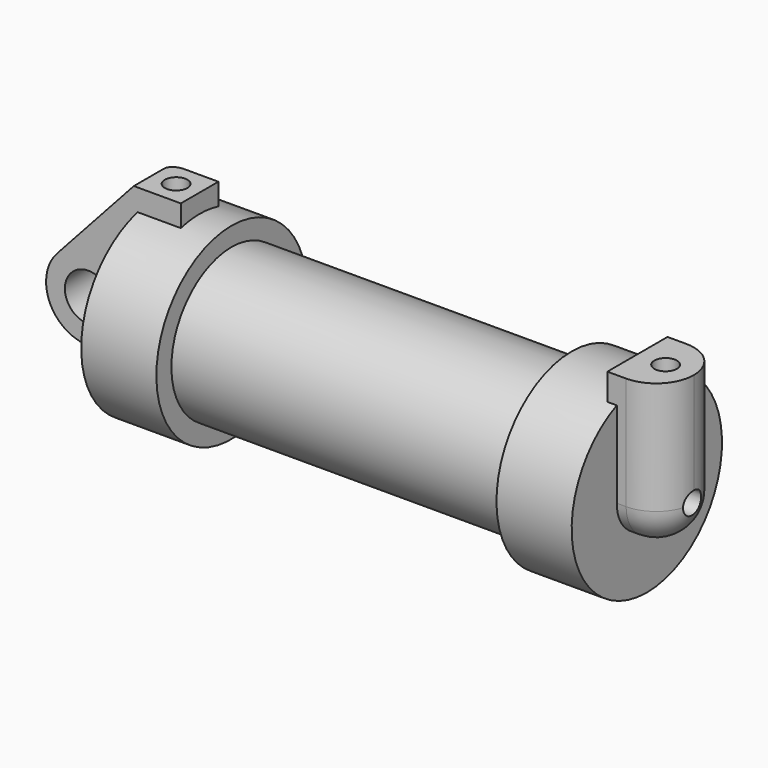
from build123d import *

# Parameters (mm, degrees)
F0_W          = 5.842
F0_H          = 12.7
F0_R          = 3.175
F2_DEPTH      = 3.175
F3_R          = 1.524
F4_DEPTH      = 6.35
F4_DEPTH_BACK = 1.27
F5_R          = 1.524
F6_DEPTH      = 10.414
F7_R          = 1.524
F8_DEPTH      = 17.78
F9_DEPTH      = 56.134
F10_R         = 1.27
F11_T1_DEPTH  = 27.94
F11_T4_ANGLE  = 180


# Not quite as in the source:
# - a fillet or chamfer that OpenCascade refuses, or shapes differently, is made with other operations: its cross-section is extruded or revolved along the edge and cut away or added


with BuildPart() as f1:
    # F0 (on Front) → F1 (revolve)
    with BuildSketch(Plane.XZ):
        Polygon((5.842, 12.7), (5.842, 0), (66.294, 0), (66.294, 12.7), (56.134, 12.7), (56.134, 10.16), (10.16, 10.16), (10.16, 12.7), align=None)
        with Locations((2.921, 6.35)):
            Rectangle(F0_W, F0_H)
    revolve(axis=Axis((33.147, 0, 0), (-1, 0, 0)))

    # F0 (on Front) → F2 (join, symmetric)
    with BuildSketch(Plane.XZ):
        with BuildLine():
            Line((-0.9398, 0), (0, 0))
            Line((0, 0), (0, 12.7))
            Line((0, 12.7), (5.842, 12.7))
            Line((5.842, 12.7), (5.842, 15.24))
            Line((5.842, 15.24), (-0.508, 15.24))
            Line((-0.508, 15.24), (-10.8806298187, 3.8475430269))
            ThreePointArc((-10.8806298187, 3.8475430269), (-4.5919612295, 5.3297205562), (-0.9398, 0))
        make_face()
        with Locations((2.921, 6.35)):
            Rectangle(F0_W, F0_H)
        with BuildLine():
            Line((5.842, 0), (0, 0))
            Line((0, 0), (-0.9398, 0))
            ThreePointArc((-0.9398, 0), (-3.1957909266, -4.5493385486), (-8.1826630726, -5.5069827884))
            Line((-8.1826630726, -5.5069827884), (5.842, -9.398))
            Line((5.842, -9.398), (5.842, 0))
        make_face()
        with BuildLine():
            ThreePointArc((-8.1826630726, -5.5069827884), (-3.1957909266, -4.5493385486), (-0.9398, 0))
            ThreePointArc((-0.9398, 0), (-4.5919612295, 5.3297205562), (-10.8806298187, 3.8475430269))
            ThreePointArc((-10.8806298187, 3.8475430269), (-12.1459778134, -1.5837270034), (-8.1826630726, -5.5069827884))
        make_face()
        with Locations((-6.6548, 0)):
            Circle(F0_R, mode=Mode.SUBTRACT)
    extrude(amount=F2_DEPTH, both=True)

    # F3 (on face) → F4 (join, two sides)
    with BuildSketch(Plane.YZ.offset(66.294)) as f4_sk:
        with BuildLine():
            ThreePointArc((-5.08, 0), (0, -5.08), (5.08, 0))
            ThreePointArc((5.08, 0), (0, 5.08), (-5.08, 0))
        make_face()
        Circle(F3_R, mode=Mode.SUBTRACT)
        with BuildLine():
            ThreePointArc((-5.08, 0), (0, 5.08), (5.08, 0))
            Line((5.08, 0), (5.08, 15.24))
            Line((5.08, 15.24), (-5.08, 15.24))
            Line((-5.08, 15.24), (-5.08, 0))
        make_face()
    extrude(amount=F4_DEPTH)
    extrude(f4_sk.sketch, amount=-F4_DEPTH_BACK)

    # F5 (on face) → F6 (cut)
    with BuildSketch(Plane.XY.offset(15.24)):
        with Locations((68.834, 0)):
            Circle(F5_R)
    extrude(amount=-F6_DEPTH, mode=Mode.SUBTRACT)

    # F7 (on face) → F8 (cut)
    with BuildSketch(Plane.XY.offset(15.24)):
        with Locations((2.667, 0)):
            Circle(F7_R)
    extrude(amount=-F8_DEPTH, mode=Mode.SUBTRACT)

    # F9 (cut, through all): a face of the model
    f9_faces = [f1.faces().sort_by_distance(p)[0] for p in [
        (66.294, 0, 0),
    ]]
    extrude(f9_faces, amount=-F9_DEPTH, mode=Mode.SUBTRACT)

    # F10
    f10_edges = [f1.edges().sort_by_distance(p)[0] for p in [
        (-12.145978, 3.175, -1.583727),
        (-5.694315, 3.175, 9.543772),
    ]]
    fillet(f10_edges, radius=F10_R)

    # F11: fillet of radius 5.08 on 2 edges, made by hand

    # F11_s2 → F11_t1 (cut)
    with BuildSketch(Plane.XY):
        with BuildLine():
            ThreePointArc((67.564, -5.08), (71.1561024484, -3.5921024484), (72.644, 0))
            Line((72.644, 0), (72.644, -5.08))
            Line((72.644, -5.08), (67.564, -5.08))
        make_face()
        with BuildLine():
            ThreePointArc((67.564, 5.08), (71.1561024484, 3.5921024484), (72.644, 0))
            Line((72.644, 0), (72.644, 5.08))
            Line((72.644, 5.08), (67.564, 5.08))
        make_face()
    extrude(amount=F11_T1_DEPTH, mode=Mode.SUBTRACT)

    # F11_s3 → F11_t4 (revolve, cut)
    with BuildSketch(Plane.XY):
        with BuildLine():
            ThreePointArc((67.564, -5.08), (71.1561024484, -3.5921024484), (72.644, 0))
            Line((72.644, 0), (72.644, -5.08))
            Line((72.644, -5.08), (67.564, -5.08))
        make_face()
    revolve(axis=Axis((72.644, 0, 0), (1, 0, 0)), revolution_arc=F11_T4_ANGLE, mode=Mode.SUBTRACT)


solid = f1.part
